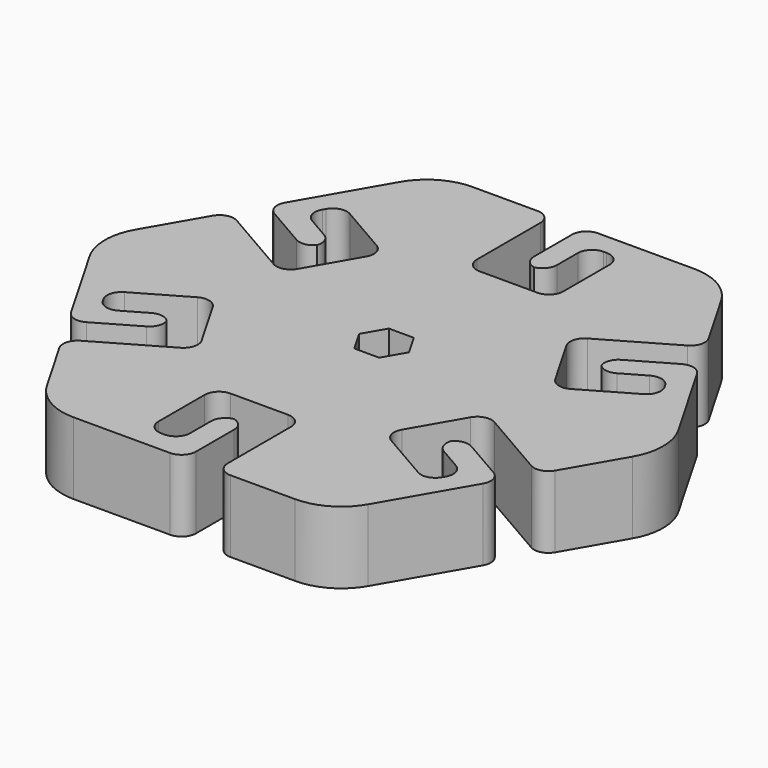
from build123d import *

# Parameters (mm, degrees)
F1_DEPTH    = 12.7
F2_R        = 10.16
F3_T1_DEPTH = 12.7
F3_T3_DEPTH = 25.4
F5_DEPTH    = 12.701


# Not quite as in the source:
# - a fillet or chamfer that OpenCascade refuses, or shapes differently, is made with other operations: its cross-section is extruded or revolved along the edge and cut away or added


with BuildPart() as f1:
    # F0 (on Top) → F1 (new body)
    with BuildSketch(Plane.XY):
        Polygon((-5.588, 24.9440905122), (-5.588, 43.9940905122), (-25.4, 43.9940905122), (-38.1, 21.9970452561), (-26.4415660143, 15.2660452561), (-24.4095660143, 18.7855724971), (-32.7684432116, 23.6115724971), (-29.9744432116, 28.4509224535), (-16.7762160579, 20.8309224535), (-24.3962160579, 7.6326952998), (-40.894, 17.1576952998), (-50.8, 0), (-38.1, -21.9970452561), (-26.4415660143, -15.2660452561), (-28.4735660143, -11.7465180151), (-36.8324432116, -16.5725180151), (-39.6264432116, -11.7331680588), (-26.4282160579, -4.1131680588), (-18.8082160579, -17.3113952125), (-35.306, -26.8363952125), (-25.4, -43.9940905122), (0, -43.9940905122), (0, -30.5320905122), (-4.064, -30.5320905122), (-4.064, -40.1840905122), (-9.652, -40.1840905122), (-9.652, -24.9440905122), (5.588, -24.9440905122), (5.588, -43.9940905122), (25.4, -43.9940905122), (38.1, -21.9970452561), (26.4415660143, -15.2660452561), (24.4095660143, -18.7855724971), (32.7684432116, -23.6115724971), (29.9744432116, -28.4509224535), (16.7762160579, -20.8309224535), (24.3962160579, -7.6326952998), (40.894, -17.1576952998), (50.8, 0), (38.1, 21.9970452561), (26.4415660143, 15.2660452561), (28.4735660143, 11.7465180151), (36.8324432116, 16.5725180151), (39.6264432116, 11.7331680588), (26.4282160579, 4.1131680588), (18.8082160579, 17.3113952125), (35.306, 26.8363952125), (25.4, 43.9940905122), (0, 43.9940905122), (0, 30.5320905122), (4.064, 30.5320905122), (4.064, 40.1840905122), (9.652, 40.1840905122), (9.652, 24.9440905122), align=None)
    extrude(amount=F1_DEPTH)

    # F2
    f2_edges = [f1.edges().sort_by_distance(p)[0] for p in [
        (-50.8, 0, 6.35),
        (-25.4, -43.994091, 6.35),
        (25.4, -43.994091, 6.35),
        (50.8, 0, 6.35),
        (25.4, 43.994091, 6.35),
        (-25.4, 43.994091, 6.35),
    ]]
    fillet(f2_edges, radius=F2_R)

    # F3: fillet of radius 2.54 on 48 edges, made by hand

    # F3_s2 → F3_t1 (join)
    with BuildSketch(Plane.XY):
        with BuildLine():
            ThreePointArc((21.0079205835, 18.5813952125), (19.8244689847, 17.0390910614), (20.0782160579, 15.1116906869))
            Line((20.0782160579, 15.1116906869), (18.8082160579, 17.3113952125))
            Line((18.8082160579, 17.3113952125), (21.0079205835, 18.5813952125))
        make_face()
        with BuildLine():
            ThreePointArc((25.1582160579, 6.3128725844), (26.700520209, 5.1294209856), (28.6279205835, 5.3831680588))
            Line((28.6279205835, 5.3831680588), (26.4282160579, 4.1131680588))
            Line((26.4282160579, 4.1131680588), (25.1582160579, 6.3128725844))
        make_face()
        with BuildLine():
            ThreePointArc((37.426738686, 10.4631680588), (38.6101902847, 12.0054722098), (38.3564432116, 13.9328725844))
            Line((38.3564432116, 13.9328725844), (39.6264432116, 11.7331680588))
            Line((39.6264432116, 11.7331680588), (37.426738686, 10.4631680588))
        make_face()
        with BuildLine():
            ThreePointArc((38.1024432116, 14.3728134895), (36.5601390605, 15.5562650883), (34.632738686, 15.3025180151))
            Line((34.632738686, 15.3025180151), (36.8324432116, 16.5725180151))
            Line((36.8324432116, 16.5725180151), (38.1024432116, 14.3728134895))
        make_face()
        with BuildLine():
            ThreePointArc((26.5959205835, -8.9026952998), (24.668520209, -8.6489482266), (23.1262160579, -9.8323998254))
            Line((23.1262160579, -9.8323998254), (24.3962160579, -7.6326952998))
            Line((24.3962160579, -7.6326952998), (26.5959205835, -8.9026952998))
        make_face()
        with BuildLine():
            ThreePointArc((18.0462160579, -18.6312179278), (17.7924689847, -20.5586183024), (18.9759205835, -22.1009224535))
            Line((18.9759205835, -22.1009224535), (16.7762160579, -20.8309224535))
            Line((16.7762160579, -20.8309224535), (18.0462160579, -18.6312179278))
        make_face()
        with BuildLine():
            ThreePointArc((27.774738686, -27.1809224535), (29.7021390605, -27.4346695266), (31.2444432116, -26.2512179278))
            Line((31.2444432116, -26.2512179278), (29.9744432116, -28.4509224535))
            Line((29.9744432116, -28.4509224535), (27.774738686, -27.1809224535))
        make_face()
        with BuildLine():
            ThreePointArc((31.4984432116, -25.8112770227), (31.7521902847, -23.8838766482), (30.568738686, -22.3415724971))
            Line((30.568738686, -22.3415724971), (32.7684432116, -23.6115724971))
            Line((32.7684432116, -23.6115724971), (31.4984432116, -25.8112770227))
        make_face()
        with BuildLine():
            ThreePointArc((5.588, -27.4840905122), (4.8440512242, -25.688039288), (3.048, -24.9440905122))
            Line((3.048, -24.9440905122), (5.588, -24.9440905122))
            Line((5.588, -24.9440905122), (5.588, -27.4840905122))
        make_face()
        with BuildLine():
            ThreePointArc((-7.112, -24.9440905122), (-8.9080512242, -25.688039288), (-9.652, -27.4840905122))
            Line((-9.652, -27.4840905122), (-9.652, -24.9440905122))
            Line((-9.652, -24.9440905122), (-7.112, -24.9440905122))
        make_face()
        with BuildLine():
            ThreePointArc((-9.652, -37.6440905122), (-8.9080512242, -39.4401417365), (-7.112, -40.1840905122))
            Line((-7.112, -40.1840905122), (-9.652, -40.1840905122))
            Line((-9.652, -40.1840905122), (-9.652, -37.6440905122))
        make_face()
        with BuildLine():
            ThreePointArc((-6.604, -40.1840905122), (-4.8079487758, -39.4401417365), (-4.064, -37.6440905122))
            Line((-4.064, -37.6440905122), (-4.064, -40.1840905122))
            Line((-4.064, -40.1840905122), (-6.604, -40.1840905122))
        make_face()
        with BuildLine():
            ThreePointArc((-20.0782160579, -15.1116906869), (-19.8244689847, -17.0390910614), (-21.0079205835, -18.5813952125))
            Line((-21.0079205835, -18.5813952125), (-18.8082160579, -17.3113952125))
            Line((-18.8082160579, -17.3113952125), (-20.0782160579, -15.1116906869))
        make_face()
        with BuildLine():
            ThreePointArc((-28.6279205835, -5.3831680588), (-26.700520209, -5.1294209856), (-25.1582160579, -6.3128725844))
            Line((-25.1582160579, -6.3128725844), (-26.4282160579, -4.1131680588))
            Line((-26.4282160579, -4.1131680588), (-28.6279205835, -5.3831680588))
        make_face()
        with BuildLine():
            ThreePointArc((-38.3564432116, -13.9328725844), (-38.6101902847, -12.0054722098), (-37.426738686, -10.4631680588))
            Line((-37.426738686, -10.4631680588), (-39.6264432116, -11.7331680588))
            Line((-39.6264432116, -11.7331680588), (-38.3564432116, -13.9328725844))
        make_face()
        with BuildLine():
            ThreePointArc((-34.632738686, -15.3025180151), (-36.5601390605, -15.5562650883), (-38.1024432116, -14.3728134895))
            Line((-38.1024432116, -14.3728134895), (-36.8324432116, -16.5725180151))
            Line((-36.8324432116, -16.5725180151), (-34.632738686, -15.3025180151))
        make_face()
        with BuildLine():
            ThreePointArc((-30.568738686, 22.3415724971), (-31.7521902847, 23.8838766482), (-31.4984432116, 25.8112770227))
            Line((-31.4984432116, 25.8112770227), (-32.7684432116, 23.6115724971))
            Line((-32.7684432116, 23.6115724971), (-30.568738686, 22.3415724971))
        make_face()
        with BuildLine():
            ThreePointArc((-23.1262160579, 9.8323998254), (-24.668520209, 8.6489482266), (-26.5959205835, 8.9026952998))
            Line((-26.5959205835, 8.9026952998), (-24.3962160579, 7.6326952998))
            Line((-24.3962160579, 7.6326952998), (-23.1262160579, 9.8323998254))
        make_face()
        with BuildLine():
            ThreePointArc((-18.9759205835, 22.1009224535), (-17.7924689847, 20.5586183024), (-18.0462160579, 18.6312179278))
            Line((-18.0462160579, 18.6312179278), (-16.7762160579, 20.8309224535))
            Line((-16.7762160579, 20.8309224535), (-18.9759205835, 22.1009224535))
        make_face()
        with BuildLine():
            ThreePointArc((-31.2444432116, 26.2512179278), (-29.7021390605, 27.4346695266), (-27.774738686, 27.1809224535))
            Line((-27.774738686, 27.1809224535), (-29.9744432116, 28.4509224535))
            Line((-29.9744432116, 28.4509224535), (-31.2444432116, 26.2512179278))
        make_face()
        with BuildLine():
            ThreePointArc((-3.048, 24.9440905122), (-4.8440512242, 25.688039288), (-5.588, 27.4840905122))
            Line((-5.588, 27.4840905122), (-5.588, 24.9440905122))
            Line((-5.588, 24.9440905122), (-3.048, 24.9440905122))
        make_face()
        with BuildLine():
            ThreePointArc((4.064, 37.6440905122), (4.8079487758, 39.4401417365), (6.604, 40.1840905122))
            Line((6.604, 40.1840905122), (4.064, 40.1840905122))
            Line((4.064, 40.1840905122), (4.064, 37.6440905122))
        make_face()
        with BuildLine():
            ThreePointArc((9.652, 27.4840905122), (8.9080512242, 25.688039288), (7.112, 24.9440905122))
            Line((7.112, 24.9440905122), (9.652, 24.9440905122))
            Line((9.652, 24.9440905122), (9.652, 27.4840905122))
        make_face()
        with BuildLine():
            ThreePointArc((7.112, 40.1840905122), (8.9080512242, 39.4401417365), (9.652, 37.6440905122))
            Line((9.652, 37.6440905122), (9.652, 40.1840905122))
            Line((9.652, 40.1840905122), (7.112, 40.1840905122))
        make_face()
    extrude(amount=F3_T1_DEPTH)

    # F3_s4 → F3_t3 (cut)
    with BuildSketch(Plane.XY.offset(-6.35)):
        with BuildLine():
            ThreePointArc((34.036, 29.0360997381), (34.2897470732, 27.1086993635), (33.1062954744, 25.5663952125))
            Line((33.1062954744, 25.5663952125), (35.306, 26.8363952125))
            Line((35.306, 26.8363952125), (34.036, 29.0360997381))
        make_face()
        with BuildLine():
            ThreePointArc((30.6732705399, 13.0165180151), (28.7458701653, 12.762770942), (27.2035660143, 13.9462225408))
            Line((27.2035660143, 13.9462225408), (28.4735660143, 11.7465180151))
            Line((28.4735660143, 11.7465180151), (30.6732705399, 13.0165180151))
        make_face()
        with BuildLine():
            ThreePointArc((27.7115660143, 13.0663407305), (27.4578189411, 14.9937411051), (28.6412705399, 16.5360452561))
            Line((28.6412705399, 16.5360452561), (26.4415660143, 15.2660452561))
            Line((26.4415660143, 15.2660452561), (27.7115660143, 13.0663407305))
        make_face()
        with BuildLine():
            ThreePointArc((35.9002954744, 20.7270452561), (37.8276958489, 20.9807923293), (39.37, 19.7973407305))
            Line((39.37, 19.7973407305), (38.1, 21.9970452561))
            Line((38.1, 21.9970452561), (35.9002954744, 20.7270452561))
        make_face()
        with BuildLine():
            ThreePointArc((42.164, -14.9579907742), (40.6216958489, -16.1414423729), (38.6942954744, -15.8876952998))
            Line((38.6942954744, -15.8876952998), (40.894, -17.1576952998))
            Line((40.894, -17.1576952998), (42.164, -14.9579907742))
        make_face()
        with BuildLine():
            ThreePointArc((35.9002954744, -20.7270452561), (37.0837470732, -22.2693494072), (36.83, -24.1967497817))
            Line((36.83, -24.1967497817), (38.1, -21.9970452561))
            Line((38.1, -21.9970452561), (35.9002954744, -20.7270452561))
        make_face()
        with BuildLine():
            ThreePointArc((25.1715660143, -17.4657497817), (26.7138701653, -16.282298183), (28.6412705399, -16.5360452561))
            Line((28.6412705399, -16.5360452561), (26.4415660143, -15.2660452561))
            Line((26.4415660143, -15.2660452561), (25.1715660143, -17.4657497817))
        make_face()
        with BuildLine():
            ThreePointArc((26.6092705399, -20.0555724971), (25.4258189411, -18.5132683461), (25.6795660143, -16.5858679715))
            Line((25.6795660143, -16.5858679715), (24.4095660143, -18.7855724971))
            Line((24.4095660143, -18.7855724971), (26.6092705399, -20.0555724971))
        make_face()
        with BuildLine():
            ThreePointArc((8.128, -43.9940905122), (6.3319487758, -43.2501417365), (5.588, -41.4540905122))
            Line((5.588, -41.4540905122), (5.588, -43.9940905122))
            Line((5.588, -43.9940905122), (8.128, -43.9940905122))
        make_face()
        with BuildLine():
            ThreePointArc((0, -41.4540905122), (-0.7439487758, -43.2501417365), (-2.54, -43.9940905122))
            Line((-2.54, -43.9940905122), (0, -43.9940905122))
            Line((0, -43.9940905122), (0, -41.4540905122))
        make_face()
        with BuildLine():
            ThreePointArc((-4.064, -33.0720905122), (-3.3200512242, -31.276039288), (-1.524, -30.5320905122))
            Line((-1.524, -30.5320905122), (-4.064, -30.5320905122))
            Line((-4.064, -30.5320905122), (-4.064, -33.0720905122))
        make_face()
        with BuildLine():
            ThreePointArc((-2.54, -30.5320905122), (-0.7439487758, -31.276039288), (0, -33.0720905122))
            Line((0, -33.0720905122), (0, -30.5320905122))
            Line((0, -30.5320905122), (-2.54, -30.5320905122))
        make_face()
        with BuildLine():
            ThreePointArc((-33.1062954744, -25.5663952125), (-34.2897470732, -27.1086993635), (-34.036, -29.0360997381))
            Line((-34.036, -29.0360997381), (-35.306, -26.8363952125))
            Line((-35.306, -26.8363952125), (-33.1062954744, -25.5663952125))
        make_face()
        with BuildLine():
            ThreePointArc((-27.2035660143, -13.9462225408), (-28.7458701653, -12.762770942), (-30.6732705399, -13.0165180151))
            Line((-30.6732705399, -13.0165180151), (-28.4735660143, -11.7465180151))
            Line((-28.4735660143, -11.7465180151), (-27.2035660143, -13.9462225408))
        make_face()
        with BuildLine():
            ThreePointArc((-28.6412705399, -16.5360452561), (-27.4578189411, -14.9937411051), (-27.7115660143, -13.0663407305))
            Line((-27.7115660143, -13.0663407305), (-26.4415660143, -15.2660452561))
            Line((-26.4415660143, -15.2660452561), (-28.6412705399, -16.5360452561))
        make_face()
        with BuildLine():
            ThreePointArc((-39.37, -19.7973407305), (-37.8276958489, -20.9807923293), (-35.9002954744, -20.7270452561))
            Line((-35.9002954744, -20.7270452561), (-38.1, -21.9970452561))
            Line((-38.1, -21.9970452561), (-39.37, -19.7973407305))
        make_face()
        with BuildLine():
            ThreePointArc((-38.6942954744, 15.8876952998), (-40.6216958489, 16.1414423729), (-42.164, 14.9579907742))
            Line((-42.164, 14.9579907742), (-40.894, 17.1576952998))
            Line((-40.894, 17.1576952998), (-38.6942954744, 15.8876952998))
        make_face()
        with BuildLine():
            ThreePointArc((-36.83, 24.1967497817), (-37.0837470732, 22.2693494072), (-35.9002954744, 20.7270452561))
            Line((-35.9002954744, 20.7270452561), (-38.1, 21.9970452561))
            Line((-38.1, 21.9970452561), (-36.83, 24.1967497817))
        make_face()
        with BuildLine():
            ThreePointArc((-28.6412705399, 16.5360452561), (-26.7138701653, 16.282298183), (-25.1715660143, 17.4657497817))
            Line((-25.1715660143, 17.4657497817), (-26.4415660143, 15.2660452561))
            Line((-26.4415660143, 15.2660452561), (-28.6412705399, 16.5360452561))
        make_face()
        with BuildLine():
            ThreePointArc((-25.6795660143, 16.5858679715), (-25.4258189411, 18.5132683461), (-26.6092705399, 20.0555724971))
            Line((-26.6092705399, 20.0555724971), (-24.4095660143, 18.7855724971))
            Line((-24.4095660143, 18.7855724971), (-25.6795660143, 16.5858679715))
        make_face()
        with BuildLine():
            ThreePointArc((-5.588, 41.4540905122), (-6.3319487758, 43.2501417365), (-8.128, 43.9940905122))
            Line((-8.128, 43.9940905122), (-5.588, 43.9940905122))
            Line((-5.588, 43.9940905122), (-5.588, 41.4540905122))
        make_face()
        with BuildLine():
            ThreePointArc((2.54, 43.9940905122), (0.7439487758, 43.2501417365), (0, 41.4540905122))
            Line((0, 41.4540905122), (0, 43.9940905122))
            Line((0, 43.9940905122), (2.54, 43.9940905122))
        make_face()
        with BuildLine():
            ThreePointArc((0, 33.0720905122), (0.7439487758, 31.276039288), (2.54, 30.5320905122))
            Line((2.54, 30.5320905122), (0, 30.5320905122))
            Line((0, 30.5320905122), (0, 33.0720905122))
        make_face()
        with BuildLine():
            ThreePointArc((1.524, 30.5320905122), (3.3200512242, 31.276039288), (4.064, 33.0720905122))
            Line((4.064, 33.0720905122), (4.064, 30.5320905122))
            Line((4.064, 30.5320905122), (1.524, 30.5320905122))
        make_face()
    extrude(amount=F3_T3_DEPTH, mode=Mode.SUBTRACT)

    # F4 (on face) → F5 (cut, through all)
    with BuildSketch(Plane.XY.offset(12.7)):
        Polygon((2.1997045256, -3.81), (4.3994090512, 0), (2.1997045256, 3.81), (-2.1997045256, 3.81), (-4.3994090512, 0), (-2.1997045256, -3.81), align=None)
    extrude(amount=-F5_DEPTH, mode=Mode.SUBTRACT)


solid = f1.part
